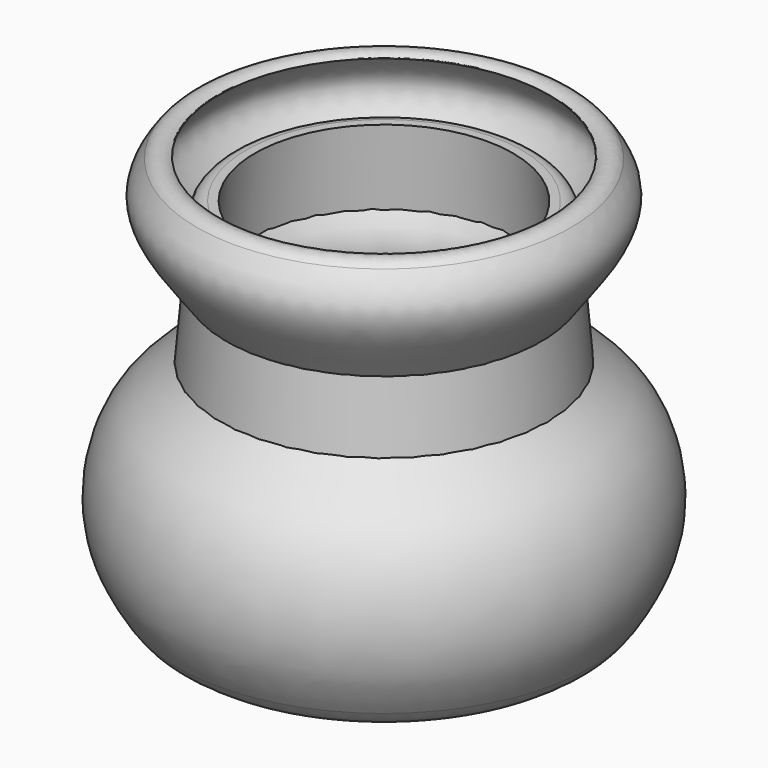
from build123d import *

# Parameters (mm, degrees)
F0_R     = 25
F1_DEPTH = 50
F1_TAPER = 5
F2_T     = -3
F3_R     = 2
F4_R     = 7
F7_R     = 7
F8_R     = 2


# Not quite as in the source:
# - ends of sketch curves that miss each other by under 0.0002 mm in the source are joined
# - the dataset's text gives a spline's control points without its knots; the knots are read off the source's solid


with BuildPart() as f1:
    # F0 (on Top) → F1 (new body)
    with BuildSketch(Plane.XY):
        Circle(F0_R)
    extrude(amount=F1_DEPTH, taper=F1_TAPER)

    # F2
    f2_openings = [f1.faces().sort_by_distance(p)[0] for p in [
        (0, 0, 50),
    ]]
    offset(amount=F2_T, openings=f2_openings)

    # F3
    f3_edges = [f1.edges().sort_by_distance(p)[0] for p in [
        (-20.625567, 0, 50),
    ]]
    fillet(f3_edges, radius=F3_R)

    # F4
    f4_edges = [f1.edges().sort_by_distance(p)[0] for p in [
        (-25, 0, 0),
    ]]
    fillet(f4_edges, radius=F4_R)


with BuildPart() as f6:
    # F5 (on Right) → F6 (revolve)
    with BuildSketch(Plane.YZ):
        with BuildLine():
            Line((2.1, 2.0999993639), (0, 2.0999993639))
            Line((0, 2.0999993639), (0, 0))
            Line((0, 0), (26.0605573531, 0))
            add(Edge.make_bspline(
                [(24.1697232449, 56.7231529161), (26.0551290778, 54.5429406989), (30.5523531052, 49.3425203983), (17.0815117654, 36.800591071), (21.2283478934, 30.8846429659), (30.9587308555, 25.149568849), (33.5055876288, 10.5447282676), (28.5213767516, 3.4853682137), (26.0605573531, 0)],
                knots=[0, 0, 0, 0, 0.1442518077, 0.3440811968, 0.4628451634, 0.6315459202, 0.8180857573, 1, 1, 1, 1], degree=3))
            Line((24.1697232449, 56.7231529161), (22.5812950581, 55.3495105959))
            add(Edge.make_bspline(
                [(22.5812950581, 55.3495105959), (22.9897400767, 54.8772001765), (23.7706969525, 53.972754158), (24.6814723031, 52.7169237229), (25.1230837979, 51.7873623848), (25.2874590889, 51.1122511584), (25.320042367, 50.6960977325), (25.3012460207, 50.3450500597), (25.2616927496, 50.0662819887), (25.192850277, 49.7675399855), (25.0847384746, 49.4232182849), (24.9374447705, 49.0434068247), (24.6898502595, 48.4956659856), (24.1295166651, 47.4470065113), (23.0261245636, 45.7735542576), (21.4454705837, 43.6435964543), (20.101366334, 41.8441250249), (19.114144807, 40.4124464453), (18.4424366998, 39.3404357899), (17.9604535555, 38.4394931704), (17.6373640956, 37.7009829924), (17.4311501496, 37.1295148001), (17.2730687275, 36.5436577418), (17.1368659625, 35.7632254815), (17.1117153283, 34.7871814502), (17.3188593508, 33.6708781977), (17.7220256738, 32.6653829285), (18.2582530643, 31.7871819258), (18.8771070407, 31.0176834707), (19.5486912207, 30.327066101), (20.487888479, 29.4767214419), (21.7374633706, 28.4752259511), (23.2844257726, 27.2860247996), (24.7994115838, 26.0541188863), (25.9663615661, 24.9600466839), (26.8044019971, 24.0299833736), (27.3774998894, 23.3015691796), (27.8873241821, 22.5376629268), (28.3508229857, 21.7085774881), (28.7619757686, 20.8274313328), (29.2377794397, 19.5918530483), (29.6902165857, 17.9554699242), (29.9914790738, 15.9148141047), (30.0431675635, 13.8699547442), (29.876907299, 12.2228342576), (29.6206529923, 10.97696407), (29.2814943641, 9.7538509383), (28.7129889766, 8.2607580834), (27.8287590901, 6.4984016536), (26.6024491617, 4.4546284909), (25.5958306642, 2.990758045), (24.9711537683, 2.1000618259)],
                knots=[0, 0, 0, 0, 0.03125, 0.0625, 0.09375, 0.109375, 0.125, 0.1328125, 0.140625, 0.1484375, 0.15625, 0.1640625, 0.171875, 0.1875, 0.21875, 0.25, 0.28125, 0.296875, 0.3125, 0.328125, 0.3359375, 0.34375, 0.3515625, 0.359375, 0.375, 0.390625, 0.40625, 0.421875, 0.4375, 0.453125, 0.46875, 0.5, 0.53125, 0.5625, 0.59375, 0.609375, 0.625, 0.640625, 0.65625, 0.671875, 0.6875, 0.71875, 0.75, 0.78125, 0.8125, 0.828125, 0.84375, 0.875, 0.90625, 0.9375, 0.9844554316, 0.9844554316, 0.9844554316, 0.9844554316], degree=3))
            Line((24.9711537683, 2.1000618259), (2.1, 2.0999993639))
        make_face()
    revolve(axis=Axis((0, 0, 30), (0, 0, -1)))

    # F7
    f7_edges = [f6.edges().sort_by_distance(p)[0] for p in [
        (0, -26.060557, 0),
    ]]
    fillet(f7_edges, radius=F7_R)

    # F8
    f8_edges = [f6.edges().sort_by_distance(p)[0] for p in [
        (0, -24.169723, 56.723153),
    ]]
    fillet(f8_edges, radius=F8_R)


solid = Compound([f1.part, f6.part])
